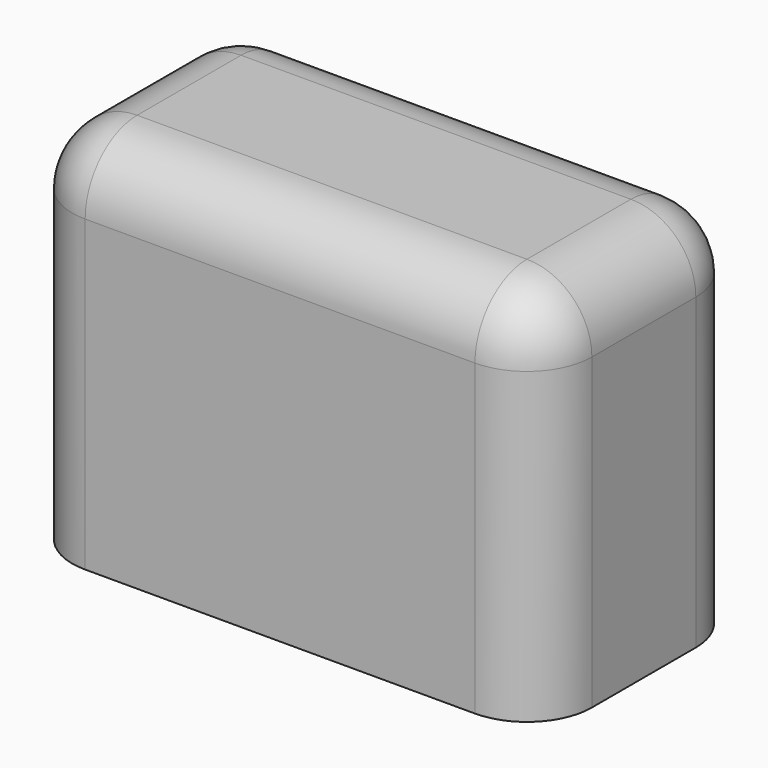
from build123d import *

# Parameters (mm, degrees)
F0_W      = 16
F0_H      = 8
F1_DEPTH  = 11.5
F2_W      = 10.2
F2_H      = 2.4
F3_DEPTH  = 8.5
F4_R      = 1.85
F5_DEPTH  = 0.5
F7_W      = 2
F7_H      = 3.7
F8_DEPTH  = 0.8
F9_SIZE2  = 3.69999
F9_SIZE   = 0.49999
F12_DEPTH = 1
F14_R     = 2


# Not quite as in the source:
# - a fillet or chamfer is up to 0.001 mm smaller than in the source, because OpenCascade refuses the exact size


with BuildPart() as f1:
    # F0 (on Top) → F1 (new body)
    with BuildSketch(Plane.XY):
        Rectangle(F0_W, F0_H)
    extrude(amount=F1_DEPTH)

    # F2 (on face) → F3 (cut)
    with BuildSketch(Plane(origin=(0, 0, 0), x_dir=(1, 0, 0), z_dir=(0, 0, -1))):
        Rectangle(F2_W, F2_H)
    extrude(amount=-F3_DEPTH, mode=Mode.SUBTRACT)

    # F14
    f14_edges = [f1.edges().sort_by_distance(p)[0] for p in [
        (0, -4, 11.5),
        (0, 4, 11.5),
        (8, 0, 11.5),
        (-8, 0, 11.5),
        (-8, -4, 5.75),
        (8, -4, 5.75),
        (8, 4, 5.75),
        (-8, 4, 5.75),
    ]]
    fillet(f14_edges, radius=F14_R)


with BuildPart() as f5:
    # F4 (on face) → F5 (new body)
    with BuildSketch(Plane.XZ.offset(-1.2)):
        with Locations((0, 3)):
            Circle(F4_R)
    extrude(amount=F5_DEPTH)


with BuildPart() as f8:
    # F7 (on face) → F8 (new body)
    with BuildSketch(Plane.XZ.offset(-1.2)):
        with Locations((0, 3)):
            Rectangle(F7_W, F7_H)
    extrude(amount=F8_DEPTH)

    # F9 (size 0.5 and 3.7 in the source; OpenCascade refuses exactly that, so slightly less here)
    f9_edges = [f8.edges().sort_by_distance(p)[0] for p in [
        (0, 0.4, 1.15),
    ]]
    f9_side = f8.faces().sort_by_distance((0, 0.8, 1.15))[0]
    chamfer(f9_edges, length=F9_SIZE, length2=F9_SIZE2, reference=f9_side)


with BuildPart() as f12:
    # F11 (on Right) → F12 (new body, symmetric)
    with BuildSketch(Plane.YZ):
        Polygon((1.2, 1.15), (1.2, 4.85), (0.7, 4.85), align=None)
    extrude(amount=F12_DEPTH, both=True)


with BuildPart() as f5_1:
    add(f5.part)

    # F13: intersect F12
    add(f12.part, mode=Mode.INTERSECT)


solid = Compound([f1.part, f5_1.part])
